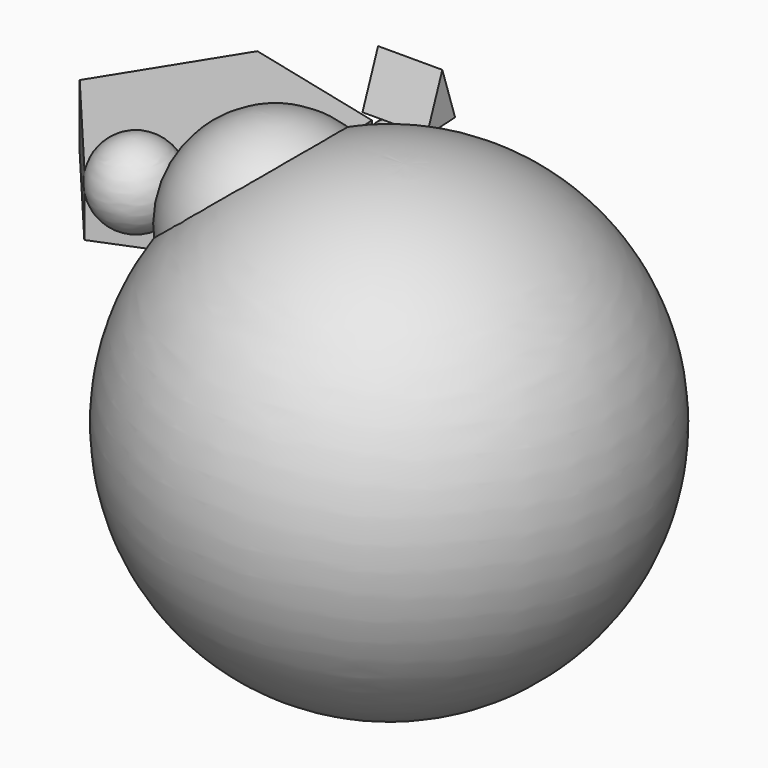
from build123d import *

# Parameters (mm, degrees)
F7_DEPTH  = 25.4
F13_DEPTH = 25.4


with BuildPart() as f1:
    # F0 (on Front) → F1 (revolve)
    with BuildSketch(Plane.XZ):
        with BuildLine():
            Line((0, -12.4185218122), (0, 62.9832169619))
            ThreePointArc((0, 62.9832169619), (-37.700869387, 25.2823475748), (0, -12.4185218122))
        make_face()
    revolve(axis=Axis((0, 0, 22.1347473562), (0, 0, -1)))


with BuildPart() as f3:
    # F2 (on Front) → F3 (revolve)
    with BuildSketch(Plane.XZ):
        with BuildLine():
            Line((-54.244944015, 6.0760609747), (-56.0079218987, 38.3973060062))
            ThreePointArc((-56.0079218987, 38.3973060062), (-71.294417695, 21.3547929726), (-54.244944015, 6.0760609747))
        make_face()
    revolve(axis=Axis((-54.7276530415, 0, 14.9257220328), (0.0544645203, 0, -0.9985157064)))


with BuildPart() as f5:
    # F4 (on Right) → F5 (revolve)
    with BuildSketch(Plane.YZ):
        with BuildLine():
            Line((55.2462321131, 25.8472459742), (55.9877101477, 38.9466989357))
            ThreePointArc((55.9877101477, 38.9466989357), (49.1920697988, 32.760645902), (55.2462321131, 25.8472459742))
        make_face()
    revolve(axis=Axis((0, 55.4384011775, 29.2422347702), (0, -0.056513279, -0.9984018476)))


with BuildPart() as f7:
    # F6 (on Right) → F7 (new body)
    with BuildSketch(Plane.YZ):
        Polygon((43.1526005268, 47.0109544694), (57.1645051241, 47.8232353926), (50.8693046868, 66.9119134545), align=None)
    extrude(amount=F7_DEPTH)


with BuildPart() as f9:
    # F8 (on Front) → F9 (revolve)
    with BuildSketch(Plane.XZ):
        with BuildLine():
            ThreePointArc((-33.2021191716, -61.3086856423), (-20.9693147125, -56.6285423392), (-15.8472371261, -44.5741005242))
            ThreePointArc((-15.8472371261, -44.5741005242), (-20.9693147125, -32.5196587092), (-33.2021191716, -27.8395154061))
            Line((-33.2021191716, -27.8395154061), (-33.2021191716, -61.3086856423))
        make_face()
    revolve(axis=Axis((-33.2021191716, 0, -46.0971305147), (0, 0, -1)))


with BuildPart() as f11:
    # F10 (on Front) → F11 (revolve)
    with BuildSketch(Plane.XZ):
        with BuildLine():
            Line((39.0098225524, -121.0559532226), (51.1082647388, 63.1703495191))
            ThreePointArc((51.1082647388, 63.1703495191), (-47.1329459571, -22.8884033231), (39.0098225524, -121.0559532226))
        make_face()
    revolve(axis=Axis((45.7032993436, 0, -19.1325433552), (-0.0655304765, 0, -0.9978505683)))


with BuildPart() as f13:
    # F12 (on Top) → F13 (new body)
    with BuildSketch(Plane.XY):
        Polygon((-20.3116302609, 73.1910519361), (-76.7818997383, 87.2138686419), (-107.5686638887, 37.8407395497), (-70.1256610599, -6.6963490662), (-16.1978485205, 15.1513455015), align=None)
    extrude(amount=F13_DEPTH)


solid = Compound([f1.part, f3.part, f5.part, f7.part, f9.part, f11.part, f13.part])
